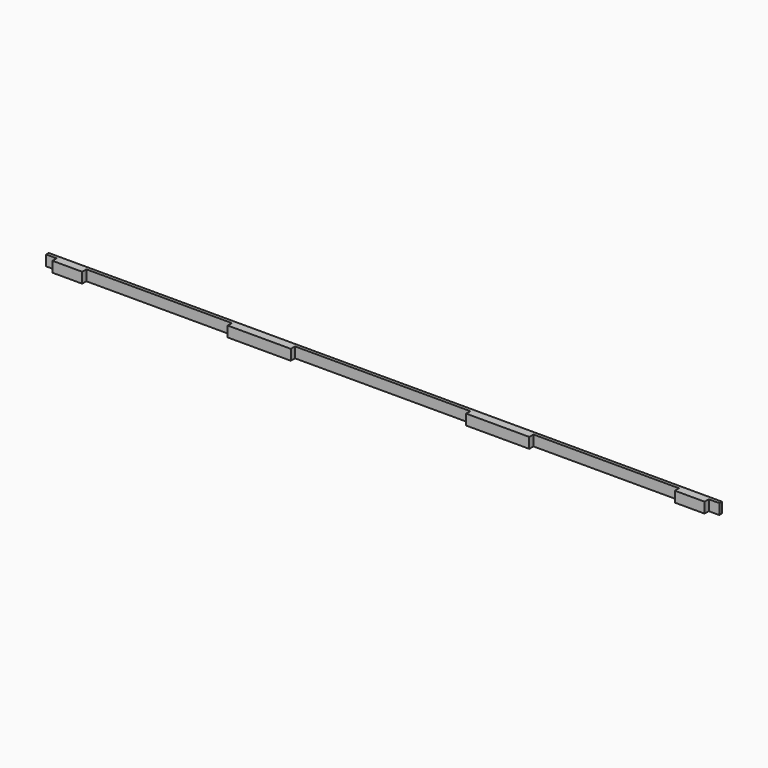
from build123d import *

# Parameters (mm, degrees)
F1_W     = 2438.4
F1_H     = 38.1
F2_DEPTH = 11.938
F3_W     = 107.95
F3_H     = 38.1
F3_W_2   = 228.6
F4_DEPTH = 19.05


# Not quite as in the source:
# - a variable given as a bare number and used for a length is read in inches; the dataset says mm whatever the document's units were


with BuildPart() as f2:
    # F1 (on Front) → F2 (new body)
    with BuildSketch(Plane.XZ):
        with Locations((1219.2, -19.05)):
            Rectangle(F1_W, F1_H)
    extrude(amount=F2_DEPTH)

    # F3 (on face) → F4 (join)
    with BuildSketch(Plane.XZ.offset(11.938)):
        with Locations((92.075, -19.05)):
            Rectangle(F3_W, F3_H)
        with Locations((2346.325, -19.05)):
            Rectangle(F3_W, F3_H)
        with Locations((787.4, -19.05)):
            Rectangle(F3_W_2, F3_H)
        with Locations((1651, -19.05)):
            Rectangle(F3_W_2, F3_H)
    extrude(amount=F4_DEPTH)


solid = f2.part
